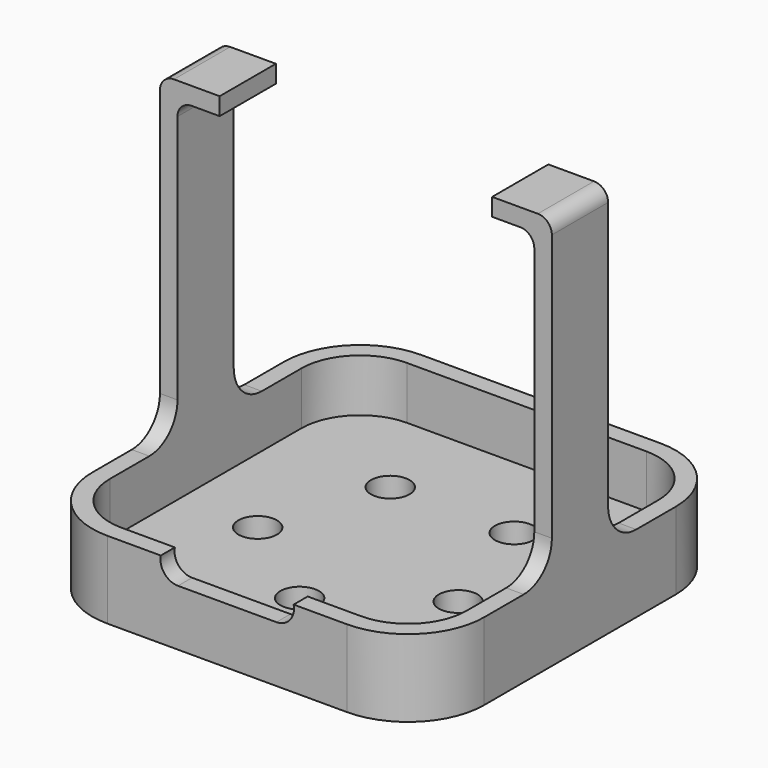
from build123d import *

# Parameters (mm, degrees)
F1_DEPTH  = 3.5
F2_DEPTH  = 11
F4_DEPTH  = 25
F5_W      = 2.5
F5_H      = 10
F6_DEPTH  = 42.5
F7_W      = 2.5
F7_H      = 10
F7_W_2    = 6
F8_DEPTH  = 2.5
F9_R      = 2
F10_R     = 5
F11_R     = 2.75
F12_DEPTH = 3.2


# Not quite as in the source:
# - a pattern or mirror of a feature is missing from the dataset's text; its kind, count and spacing are read off the source's solid


with BuildPart() as f1:
    # F0 (on Top) → F1 (new body)
    with BuildSketch(Plane.XY):
        with BuildLine():
            ThreePointArc((25.385, 17.035), (22.9393416229, 22.9393416229), (17.035, 25.385))
            Line((17.035, 25.385), (-17.035, 25.385))
            ThreePointArc((-17.035, 25.385), (-22.9393416229, 22.9393416229), (-25.385, 17.035))
            Line((-25.385, 17.035), (-25.385, -17.035))
            ThreePointArc((-25.385, -17.035), (-22.9393416229, -22.9393416229), (-17.035, -25.385))
            Line((-17.035, -25.385), (17.035, -25.385))
            ThreePointArc((17.035, -25.385), (22.9393416229, -22.9393416229), (25.385, -17.035))
            Line((25.385, -17.035), (25.385, 17.035))
        make_face()
    extrude(amount=F1_DEPTH)

    # F0 (on Top) → F2 (join)
    with BuildSketch(Plane.XY):
        with BuildLine():
            ThreePointArc((27.885, 17.035), (24.7071085759, 24.7071085759), (17.035, 27.885))
            Line((17.035, 27.885), (-17.035, 27.885))
            ThreePointArc((-17.035, 27.885), (-24.7071085759, 24.7071085759), (-27.885, 17.035))
            Line((-27.885, 17.035), (-27.885, -17.035))
            ThreePointArc((-27.885, -17.035), (-24.7071085759, -24.7071085759), (-17.035, -27.885))
            Line((-17.035, -27.885), (17.035, -27.885))
            ThreePointArc((17.035, -27.885), (24.7071085759, -24.7071085759), (27.885, -17.035))
            Line((27.885, -17.035), (27.885, 17.035))
        make_face()
        with BuildLine():
            Line((-17.035, 25.385), (17.035, 25.385))
            ThreePointArc((17.035, 25.385), (22.9393416229, 22.9393416229), (25.385, 17.035))
            Line((25.385, 17.035), (25.385, -17.035))
            ThreePointArc((25.385, -17.035), (22.9393416229, -22.9393416229), (17.035, -25.385))
            Line((17.035, -25.385), (-17.035, -25.385))
            ThreePointArc((-17.035, -25.385), (-22.9393416229, -22.9393416229), (-25.385, -17.035))
            Line((-25.385, -17.035), (-25.385, 17.035))
            ThreePointArc((-25.385, 17.035), (-22.9393416229, 22.9393416229), (-17.035, 25.385))
        make_face(mode=Mode.SUBTRACT)
    extrude(amount=F2_DEPTH)

    # F3 (on face) → F4 (cut)
    with BuildSketch(Plane.XZ.offset(27.885)):
        with BuildLine():
            ThreePointArc((-9.4494897428, 11), (-8.9364916731, 8.9188611699), (-7, 8))
            Line((-7, 8), (7, 8))
            ThreePointArc((7, 8), (8.9364916731, 8.9188611699), (9.4494897428, 11))
            Line((9.4494897428, 11), (-9.4494897428, 11))
        make_face()
        with BuildLine():
            ThreePointArc((-7, 13), (-8.5811388301, 12.4364916731), (-9.4494897428, 11))
            Line((-9.4494897428, 11), (9.4494897428, 11))
            ThreePointArc((9.4494897428, 11), (8.5811388301, 12.4364916731), (7, 13))
            Line((7, 13), (-7, 13))
        make_face()
    extrude(amount=-F4_DEPTH, mode=Mode.SUBTRACT)

    # F5 (on face) → F6 (join)
    with BuildSketch(Plane.XY.offset(11)):
        with Locations((26.635, 0)):
            Rectangle(F5_W, F5_H)
    f6 = extrude(amount=F6_DEPTH)

    # F6_copies: F6 across plane
    add(f6.mirror(Plane(origin=(0, 0, 0), x_dir=(0, 0, -1), z_dir=(-1, 0, 0))))

    # F7 (on face) → F8 (join)
    with BuildSketch(Plane.XY.offset(53.5)):
        with Locations((26.635, 0)):
            Rectangle(F7_W, F7_H)
        with Locations((22.385, 0)):
            Rectangle(F7_W_2, F7_H)
    f8 = extrude(amount=F8_DEPTH)

    # F8_copies: F8 across plane
    add(f8.mirror(Plane(origin=(0, 0, 0), x_dir=(0, 0, -1), z_dir=(-1, 0, 0))))

    # F9
    f9_edges = [f1.edges().sort_by_distance(p)[0] for p in [
        (25.385, 0, 53.5),
        (27.885, 0, 56),
        (-25.385, 0, 53.5),
        (-27.885, 0, 56),
    ]]
    fillet(f9_edges, radius=F9_R)

    # F10
    f10_edges = [f1.edges().sort_by_distance(p)[0] for p in [
        (26.635, 5, 11),
        (26.635, -5, 11),
        (-26.635, 5, 11),
        (-26.635, -5, 11),
    ]]
    fillet(f10_edges, radius=F10_R)

    # F11 (on face) → F12 (cut)
    with BuildSketch(Plane.XY.offset(3.5)):
        with Locations((0, -15)):
            Circle(F11_R)
        with Locations((14.2658477444, -4.6352549156)):
            Circle(F11_R)
        with Locations((8.8167787844, 12.1352549156)):
            Circle(F11_R)
        with Locations((-8.8167787844, 12.1352549156)):
            Circle(F11_R)
        with Locations((-14.2658477444, -4.6352549156)):
            Circle(F11_R)
    extrude(amount=-F12_DEPTH, mode=Mode.SUBTRACT)


solid = f1.part
